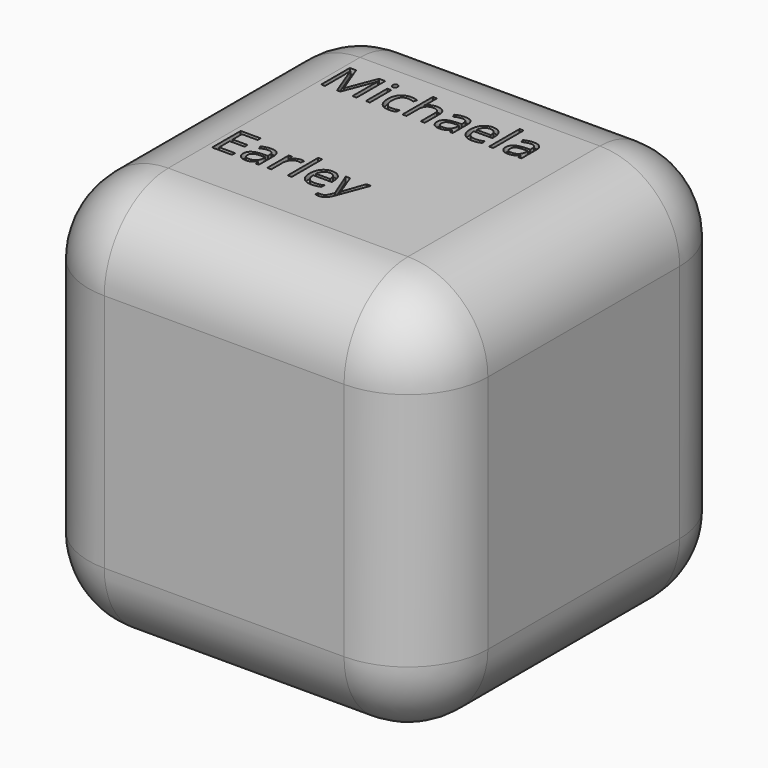
from build123d import *

# Parameters (mm, degrees)
F0_W         = 25.4
F0_H         = 25.4
F1_DEPTH     = 25.4
F2_R         = 5.08
F3_T1_DEPTH  = 33.02
F3_S5_W      = 5.08
F3_S5_H      = 5.08
F3_T6_DEPTH  = 5.08
F3_S11_W     = 5.08
F3_S11_H     = 5.08
F3_T12_DEPTH = 5.08
F4_R         = 5.08
F5_TEXT_SIZE = 3.1867245626
F6_DEPTH     = 0.3175


# Not quite as in the source:
# - a fillet or chamfer that OpenCascade refuses, or shapes differently, is made with other operations: its cross-section is extruded or revolved along the edge and cut away or added
# - Text() gives the source's letters only with a copy of the font that has no kerning and outlines rounded to 1/6400 em; it was checked with that copy


with BuildPart() as f1:
    # F0 (on Top) → F1 (new body)
    with BuildSketch(Plane.XY):
        with Locations((6.7932211466, 19.1409621991)):
            Rectangle(F0_W, F0_H)
    extrude(amount=F1_DEPTH)

    # F2
    f2_edges = [f1.edges().sort_by_distance(p)[0] for p in [
        (-5.906779, 19.140962, 25.4),
        (6.793221, 31.840962, 25.4),
        (-5.906779, 31.840962, 12.7),
        (6.793221, 31.840962, 0),
        (19.493221, 31.840962, 12.7),
        (19.493221, 19.140962, 0),
    ]]
    fillet(f2_edges, radius=F2_R)

    # F3: fillet of radius 5.08 on 3 edges, made by hand

    # F3_s2 → F3_t1 (cut)
    with BuildSketch(Plane.XZ.offset(-26.7609621991)):
        with BuildLine():
            ThreePointArc((14.4132211466, 25.4), (18.005323595, 23.9121024484), (19.4932211466, 20.32))
            Line((19.4932211466, 20.32), (19.4932211466, 25.4))
            Line((19.4932211466, 25.4), (14.4132211466, 25.4))
        make_face()
        with BuildLine():
            ThreePointArc((-5.9067788534, 5.08), (-4.4188813018, 1.4878975516), (-0.8267788534, 0))
            Line((-0.8267788534, 0), (-5.9067788534, 0))
            Line((-5.9067788534, 0), (-5.9067788534, 5.08))
        make_face()
    extrude(amount=F3_T1_DEPTH, mode=Mode.SUBTRACT)


with BuildPart() as f3_tool4:
    # F3_s5 → F3_t6 (new body)
    with BuildSketch(Plane.YZ.offset(-0.8267788534)):
        with Locations((29.3009621991, 2.54)):
            Rectangle(F3_S5_W, F3_S5_H)
    extrude(amount=-F3_T6_DEPTH)

    # F3_s7 → F3_t8 (revolve, cut)
    with BuildSketch(Plane(origin=(-0.8267788534, 26.7609621991, 5.08), x_dir=(0, -0.7071067812, 0.7071067812), z_dir=(0, -0.7071067812, -0.7071067812))):
        with BuildLine():
            ThreePointArc((0, -5.08), (5.08, 0), (0, 5.08))
            Line((0, 5.08), (0, -5.08))
        make_face()
    revolve(axis=Axis((-0.8267788534, 26.7609621991, 5.08), (-1, 0, 0)), mode=Mode.SUBTRACT)


with BuildPart() as f1_1:
    add(f1.part)

    # F3_t3: cut F3_tool4
    add(f3_tool4.part, mode=Mode.SUBTRACT)


with BuildPart() as f3_tool10:
    # F3_s11 → F3_t12 (new body)
    with BuildSketch(Plane.XY.offset(20.32)):
        with Locations((16.9532211466, 29.3009621991)):
            Rectangle(F3_S11_W, F3_S11_H)
    extrude(amount=F3_T12_DEPTH)

    # F3_s13 → F3_t14 (revolve, cut)
    with BuildSketch(Plane(origin=(14.4132211466, 26.7609621991, 20.32), x_dir=(-0.7071067812, -0.7071067812, 0), z_dir=(-0.7071067812, 0.7071067812, 0))):
        with BuildLine():
            ThreePointArc((0, -5.08), (5.08, 0), (0, 5.08))
            Line((0, 5.08), (0, -5.08))
        make_face()
    revolve(axis=Axis((14.4132211466, 26.7609621991, 20.32), (0, 0, 1)), mode=Mode.SUBTRACT)


with BuildPart() as f1_2:
    add(f1_1.part)

    # F3_t9: cut F3_tool10
    add(f3_tool10.part, mode=Mode.SUBTRACT)

    # F4
    f4_edges = [f1_2.edges().sort_by_distance(p)[0] for p in [
        (6.793221, 6.440962, 0),
    ]]
    fillet(f4_edges, radius=F4_R)

    # F5 (on face) → F6 (cut)
    with BuildSketch(Plane.XY.offset(25.4)):
        with Locations((-0.8267788534, 23.2834089547)):
            Text('Michaela', F5_TEXT_SIZE, font='Open Sans', text_align=(TextAlign.LEFT, TextAlign.BOTTOM))
        with Locations((-0.8267788534, 14.6155181444)):
            Text('Earley', F5_TEXT_SIZE, font='Open Sans', text_align=(TextAlign.LEFT, TextAlign.BOTTOM))
    extrude(amount=-F6_DEPTH, mode=Mode.SUBTRACT)


solid = f1_2.part
